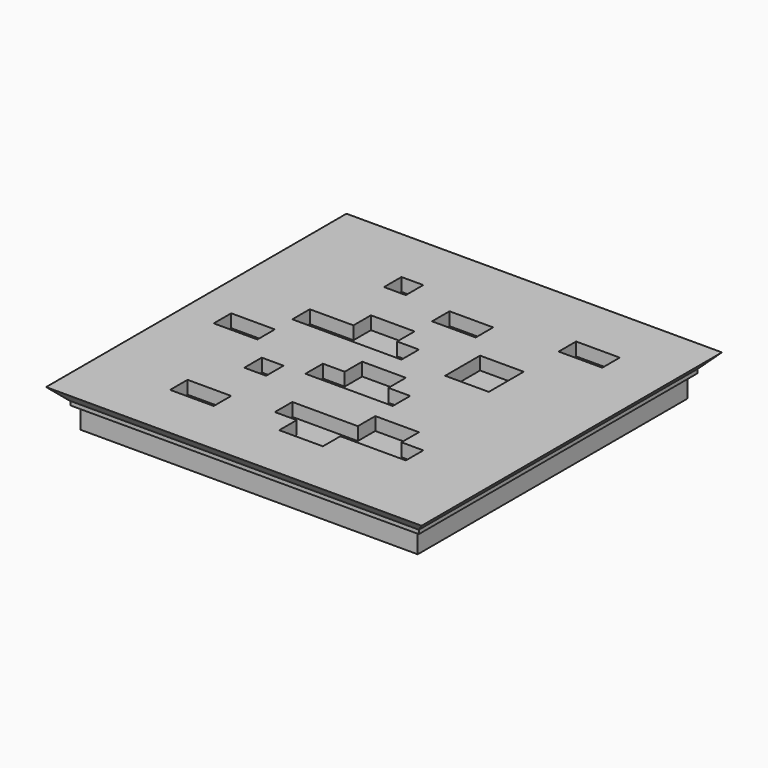
from build123d import *

# Parameters (mm, degrees)
F0_W      = 77.25
F0_H      = 77.25
F0_W_2    = 73.25
F0_H_2    = 73.25
F1_DEPTH  = 5
F2_W      = 79.8
F2_H      = 79.8
F2_W_2    = 77.25
F2_H_2    = 77.25
F2_W_3    = 73.25
F2_H_3    = 73.25
F3_DEPTH  = 0.96
F4_R      = 5
F5_DEPTH  = 5.96
F6_W      = 86
F6_H      = 86
F7_DEPTH  = 3
F8_R      = 4.9
F9_DEPTH  = 1
F10_W     = 10
F10_H     = 5
F10_W_2   = 5
F10_H_2   = 10
F11_DEPTH = 25
F20_DEPTH = 86
F21_DEPTH = 86
F22_DEPTH = 86.001
F23_REACH = 90.2436406871


with BuildPart() as f1:
    # F0 (on Top) → F1 (new body)
    with BuildSketch(Plane.XY):
        Rectangle(F0_W, F0_H)
        Rectangle(F0_W_2, F0_H_2, mode=Mode.SUBTRACT)
    extrude(amount=F1_DEPTH)

    # F2 (on face) → F3 (join)
    with BuildSketch(Plane.XY.offset(5)):
        Rectangle(F2_W, F2_H)
        Rectangle(F2_W_2, F2_H_2, mode=Mode.SUBTRACT)
        Rectangle(F2_W_2, F2_H_2)
        Rectangle(F2_W_3, F2_H_3, mode=Mode.SUBTRACT)
        Rectangle(F2_W_3, F2_H_3)
    extrude(amount=F3_DEPTH)

    # F4 (on face) → F5 (cut, through all)
    with BuildSketch(Plane.XY.offset(5.96)):
        with Locations((-31.1867402621, -16.7084898855)):
            Circle(F4_R)
        with Locations((-27.9344634459, 20.4642405513)):
            Circle(F4_R)
        with Locations((22.7069496598, -5.9243687574)):
            Circle(F4_R)
    extrude(amount=-F5_DEPTH, mode=Mode.SUBTRACT)


with BuildPart() as f7:
    # F6 (on face) → F7 (new body)
    with BuildSketch(Plane.XY.offset(5.96)):
        Rectangle(F6_W, F6_H)
    extrude(amount=F7_DEPTH)

    # F8 (on face) → F9 (join)
    with BuildSketch(Plane.XY.offset(5.96)):
        with Locations((-31.1867402621, -16.7084898855)):
            Circle(F8_R)
        with Locations((22.7069496598, -5.9243687574)):
            Circle(F8_R)
        with Locations((-27.9344634459, 20.4642405513)):
            Circle(F8_R)
    extrude(amount=-F9_DEPTH)

    # F10 (on face) → F11 (cut)
    with BuildSketch(Plane.XY.offset(8.96)):
        with Locations((-20, -27.5)):
            Rectangle(F10_W, F10_H)
        Polygon((20, -15), (10, -15), (10, -20), (-5, -20), (-5, -25), (0, -25), (0, -30), (10, -30), (10, -25), (25, -25), (25, -20), (20, -20), align=None)
        Polygon((5, -5), (5, 0), (-5, 0), (-5, -5), (-10, -5), (-10, -10), (10, -10), (10, -5), align=None)
        with Locations((-17.5, -12.5)):
            Rectangle(F10_W_2, F10_H)
        with Locations((-30, -2.5)):
            Rectangle(F10_W, F10_H)
        with Locations((-17.5, 27.5)):
            Rectangle(F10_W_2, F10_H)
        with Locations((0, 22.5)):
            Rectangle(F10_W, F10_H)
        with Locations((15, 10)):
            Rectangle(F10_W, F10_H_2)
        with Locations((25, 27.5)):
            Rectangle(F10_W, F10_H)
        Polygon((-25, 5), (0, 5), (0, 10), (-5, 10), (-5, 15), (-15, 15), (-15, 10), (-25, 10), align=None)
    extrude(amount=-F11_DEPTH, mode=Mode.SUBTRACT)

    # F16 (on offset) → F20 (cut, through all)
    with BuildSketch(Plane.XZ.offset(43)):
        Polygon((-43, 8.96), (-43, 5.96), (-40, 5.96), align=None)
    extrude(amount=-F20_DEPTH, mode=Mode.SUBTRACT)

    # F17 (on offset) → F21 (cut, through all)
    with BuildSketch(Plane(origin=(-43, 0, 0), x_dir=(0, -1, 0), z_dir=(-1, 0, 0))):
        Polygon((43, 5.96), (43, 8.96), (40, 5.96), align=None)
    extrude(amount=-F21_DEPTH, mode=Mode.SUBTRACT)

    # F18 (on offset) → F22 (cut, through all)
    with BuildSketch(Plane(origin=(0, 43, 0), x_dir=(-1, 0, 0), z_dir=(0, 1, 0))):
        Polygon((-40, 5.96), (-43, 8.96), (-43, 5.96), align=None)
    extrude(amount=-F22_DEPTH, mode=Mode.SUBTRACT)

    f23_end = f7.faces().sort_by_distance((-41.5088757396, 0.7455621302, 7.4688757396))[0]
    # F19 (on offset) → F23 (cut, up to a face of the model that its end follows)
    with BuildSketch(Plane.YZ.offset(43)):
        Polygon((43, 5.96), (43, 8.96), (40, 5.96), align=None)
    f23_long = extrude(amount=-F23_REACH, mode=Mode.PRIVATE)
    add(split(f23_long, bisect_by=f23_end, keep=Keep.BOTTOM, mode=Mode.PRIVATE), mode=Mode.SUBTRACT)


solid = Compound([f1.part, f7.part])
